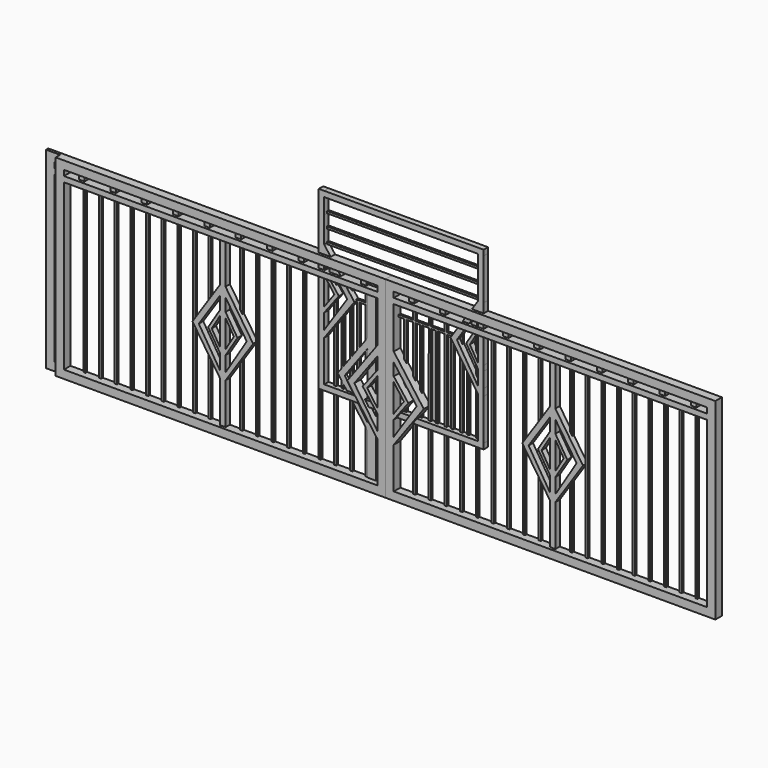
from build123d import *

# Parameters (mm, degrees)
F1_DEPTH  = 76.2
F2_DEPTH  = 25.4
F0_W      = 3048
F0_H      = 1778
F0_W_2    = 50.8
F0_H_2    = 50.8
F3_DEPTH  = 50.8
F4_DEPTH  = 50.8
F0_W_3    = 19.05
F0_H_3    = 1524
F5_DEPTH  = 19.05
F5_TAPER  = -3
F8_DEPTH  = 50.8
F9_DEPTH  = 19.05
F10_DEPTH = 19.05


with BuildPart() as f1:
    # F0 (on Front) → F1 (new body)
    with BuildSketch(Plane.XZ):
        Polygon((3048, 0), (0, 0), (0, -127), (0, -1778), (3048, -1778), align=None)
        Polygon((288.1671190262, -939.8), (76.2, -1257.9814855576), (76.2, -1117.6593963623), (210.9978, -939.8), (76.2, -765.7700244904), (76.2, -652.1689665667), align=None, mode=Mode.SUBTRACT)
        Polygon((76.2, -1069.802350235), (76.2, -813.0455196381), (170.0328290463, -939.8), align=None, mode=Mode.SUBTRACT)
        Polygon((210.9978, -1701.8), (76.2, -1701.8), (76.2, -1322.4239349365), (210.9978, -1137.1291241641), (230.0478, -1110.9427461578), (353.8880646229, -940.7103061676), (230.0478, -772.6639437989), (210.9978, -746.8138439717), (76.2, -563.8985375947), (76.2, -177.8), (210.9978, -177.8), (230.0478, -177.8), (355.7778, -177.8), (374.8278, -177.8), (500.5578, -177.8), (519.6078, -177.8), (645.3378, -177.8), (664.3878, -177.8), (790.1178, -177.8), (809.1678, -177.8), (934.8978, -177.8), (953.9478, -177.8), (1079.6778, -177.8), (1098.7278, -177.8), (1224.4578, -177.8), (1243.5078, -177.8), (1369.2378, -177.8), (1388.2878, -177.8), (1498.6, -177.8), (1549.4, -177.8), (1659.7122, -177.8), (1678.7622, -177.8), (1804.4922, -177.8), (1823.5422, -177.8), (1949.2722, -177.8), (1968.3222, -177.8), (2094.0522, -177.8), (2113.1022, -177.8), (2238.8322, -177.8), (2257.8822, -177.8), (2383.6122, -177.8), (2402.6622, -177.8), (2528.3922, -177.8), (2547.4422, -177.8), (2673.1722, -177.8), (2692.2222, -177.8), (2817.9522, -177.8), (2837.0022, -177.8), (2971.8, -177.8), (2971.8, -1701.8), (2837.0022, -1701.8), (2817.9522, -1701.8), (2692.2222, -1701.8), (2673.1722, -1701.8), (2547.4422, -1701.8), (2528.3922, -1701.8), (2402.6622, -1701.8), (2383.6122, -1701.8), (2257.8822, -1701.8), (2238.8322, -1701.8), (2113.1022, -1701.8), (2094.0522, -1701.8), (1968.3222, -1701.8), (1949.2722, -1701.8), (1823.5422, -1701.8), (1804.4922, -1701.8), (1678.7622, -1701.8), (1659.7122, -1701.8), (1549.4, -1701.8), (1498.6, -1701.8), (1388.2878, -1701.8), (1369.2378, -1701.8), (1243.5078, -1701.8), (1224.4578, -1701.8), (1098.7278, -1701.8), (1079.6778, -1701.8), (953.9478, -1701.8), (934.8978, -1701.8), (809.1678, -1701.8), (790.1178, -1701.8), (664.3878, -1701.8), (645.3378, -1701.8), (519.6078, -1701.8), (500.5578, -1701.8), (374.8278, -1701.8), (352.0028389181, -1701.8), (230.0478, -1701.8), align=None, mode=Mode.SUBTRACT)
        Polygon((196.0372, -127), (76.2, -127), (76.2, -76.2), (196.0372, -76.2), (246.8372, -76.2), (485.5972, -76.2), (536.3972, -76.2), (775.1572, -76.2), (825.9572, -76.2), (1064.7172, -76.2), (1115.5172, -76.2), (1354.2772, -76.2), (1405.0772, -76.2), (1643.8372, -76.2), (1694.6372, -76.2), (1933.3972, -76.2), (1984.1972, -76.2), (2222.9572, -76.2), (2273.7572, -76.2), (2512.5172, -76.2), (2563.3172, -76.2), (2802.0772, -76.2), (2852.8772, -76.2), (2971.8, -76.2), (2971.8, -127), (2852.8772, -127), (2802.0772, -127), (2563.3172, -127), (2512.5172, -127), (2273.7572, -127), (2222.9572, -127), (1984.1972, -127), (1933.3972, -127), (1694.6372, -127), (1643.8372, -127), (1405.0772, -127), (1354.2772, -127), (1115.5172, -127), (1064.7172, -127), (825.9572, -127), (775.1572, -127), (536.3972, -127), (485.5972, -127), (246.8372, -127), align=None, mode=Mode.SUBTRACT)
    extrude(amount=F1_DEPTH)

    # F0 (on Front) → F2 (join)
    with BuildSketch(Plane.XZ):
        Polygon((3048, 0), (0, 0), (0, -127), (0, -1778), (3048, -1778), align=None)
        Polygon((288.1671190262, -939.8), (76.2, -1257.9814855576), (76.2, -1117.6593963623), (210.9978, -939.8), (76.2, -765.7700244904), (76.2, -652.1689665667), align=None, mode=Mode.SUBTRACT)
        Polygon((76.2, -1069.802350235), (76.2, -813.0455196381), (170.0328290463, -939.8), align=None, mode=Mode.SUBTRACT)
        Polygon((210.9978, -1701.8), (76.2, -1701.8), (76.2, -1322.4239349365), (210.9978, -1137.1291241641), (230.0478, -1110.9427461578), (353.8880646229, -940.7103061676), (230.0478, -772.6639437989), (210.9978, -746.8138439717), (76.2, -563.8985375947), (76.2, -177.8), (210.9978, -177.8), (230.0478, -177.8), (355.7778, -177.8), (374.8278, -177.8), (500.5578, -177.8), (519.6078, -177.8), (645.3378, -177.8), (664.3878, -177.8), (790.1178, -177.8), (809.1678, -177.8), (934.8978, -177.8), (953.9478, -177.8), (1079.6778, -177.8), (1098.7278, -177.8), (1224.4578, -177.8), (1243.5078, -177.8), (1369.2378, -177.8), (1388.2878, -177.8), (1498.6, -177.8), (1549.4, -177.8), (1659.7122, -177.8), (1678.7622, -177.8), (1804.4922, -177.8), (1823.5422, -177.8), (1949.2722, -177.8), (1968.3222, -177.8), (2094.0522, -177.8), (2113.1022, -177.8), (2238.8322, -177.8), (2257.8822, -177.8), (2383.6122, -177.8), (2402.6622, -177.8), (2528.3922, -177.8), (2547.4422, -177.8), (2673.1722, -177.8), (2692.2222, -177.8), (2817.9522, -177.8), (2837.0022, -177.8), (2971.8, -177.8), (2971.8, -1701.8), (2837.0022, -1701.8), (2817.9522, -1701.8), (2692.2222, -1701.8), (2673.1722, -1701.8), (2547.4422, -1701.8), (2528.3922, -1701.8), (2402.6622, -1701.8), (2383.6122, -1701.8), (2257.8822, -1701.8), (2238.8322, -1701.8), (2113.1022, -1701.8), (2094.0522, -1701.8), (1968.3222, -1701.8), (1949.2722, -1701.8), (1823.5422, -1701.8), (1804.4922, -1701.8), (1678.7622, -1701.8), (1659.7122, -1701.8), (1549.4, -1701.8), (1498.6, -1701.8), (1388.2878, -1701.8), (1369.2378, -1701.8), (1243.5078, -1701.8), (1224.4578, -1701.8), (1098.7278, -1701.8), (1079.6778, -1701.8), (953.9478, -1701.8), (934.8978, -1701.8), (809.1678, -1701.8), (790.1178, -1701.8), (664.3878, -1701.8), (645.3378, -1701.8), (519.6078, -1701.8), (500.5578, -1701.8), (374.8278, -1701.8), (352.0028389181, -1701.8), (230.0478, -1701.8), align=None, mode=Mode.SUBTRACT)
        Polygon((196.0372, -127), (76.2, -127), (76.2, -76.2), (196.0372, -76.2), (246.8372, -76.2), (485.5972, -76.2), (536.3972, -76.2), (775.1572, -76.2), (825.9572, -76.2), (1064.7172, -76.2), (1115.5172, -76.2), (1354.2772, -76.2), (1405.0772, -76.2), (1643.8372, -76.2), (1694.6372, -76.2), (1933.3972, -76.2), (1984.1972, -76.2), (2222.9572, -76.2), (2273.7572, -76.2), (2512.5172, -76.2), (2563.3172, -76.2), (2802.0772, -76.2), (2852.8772, -76.2), (2971.8, -76.2), (2971.8, -127), (2852.8772, -127), (2802.0772, -127), (2563.3172, -127), (2512.5172, -127), (2273.7572, -127), (2222.9572, -127), (1984.1972, -127), (1933.3972, -127), (1694.6372, -127), (1643.8372, -127), (1405.0772, -127), (1354.2772, -127), (1115.5172, -127), (1064.7172, -127), (825.9572, -127), (775.1572, -127), (536.3972, -127), (485.5972, -127), (246.8372, -127), align=None, mode=Mode.SUBTRACT)
    extrude(amount=F2_DEPTH)

    # F0 (on Front) → F3 (join)
    with BuildSketch(Plane.XZ):
        with Locations((221.4372, -101.6)):
            Rectangle(F0_W_2, F0_H_2)
        with Locations((510.9972, -101.6)):
            Rectangle(F0_W_2, F0_H_2)
        with Locations((800.5572, -101.6)):
            Rectangle(F0_W_2, F0_H_2)
        with Locations((1090.1172, -101.6)):
            Rectangle(F0_W_2, F0_H_2)
        with Locations((1379.6772, -101.6)):
            Rectangle(F0_W_2, F0_H_2)
        with Locations((1669.2372, -101.6)):
            Rectangle(F0_W_2, F0_H_2)
        with Locations((1958.7972, -101.6)):
            Rectangle(F0_W_2, F0_H_2)
        with Locations((2248.3572, -101.6)):
            Rectangle(F0_W_2, F0_H_2)
        with Locations((2537.9172, -101.6)):
            Rectangle(F0_W_2, F0_H_2)
        with Locations((2827.4772, -101.6)):
            Rectangle(F0_W_2, F0_H_2)
    extrude(amount=F3_DEPTH)

    # F0 (on Front) → F4 (join)
    with BuildSketch(Plane.XZ):
        Polygon((1369.2378, -752.0124863089), (1243.5078, -939.8), (1369.2378, -1127.5875136911), (1388.2878, -1156.0401672807), (1498.6, -1320.8), (1498.6, -1701.8), (1549.4, -1701.8), (1549.4, -1320.8), (1659.7122, -1156.0401672807), (1678.7622, -1127.5875136911), (1804.4922, -939.8), (1678.7622, -752.0124863089), (1659.7122, -723.5598327193), (1549.4, -558.8), (1549.4, -177.8), (1498.6, -177.8), (1498.6, -558.8), (1388.2878, -723.5598327193), align=None)
        Polygon((1498.6, -764.1460895538), (1388.2878, -939.8), (1498.6, -1116.0354614258), (1498.6, -1256.357550621), (1302.3867738062, -939.8), (1498.6, -646.7403173447), align=None, mode=Mode.SUBTRACT)
        Polygon((1498.6, -1068.1784152985), (1421.8034963608, -939.8), (1498.6, -811.4215847015), align=None, mode=Mode.SUBTRACT)
        Polygon((1549.4, -764.1460895538), (1549.4, -646.7403173447), (1745.6132261938, -939.8), (1549.4, -1256.357550621), (1549.4, -1116.0354614258), (1659.7122, -939.8), align=None, mode=Mode.SUBTRACT)
        Polygon((1549.4, -1068.1784152985), (1549.4, -811.4215847015), (1626.1965036392, -939.8), align=None, mode=Mode.SUBTRACT)
    extrude(amount=F4_DEPTH)

    # F0 (on Front) → F5 (join)
    with BuildSketch(Plane.XZ):
        Polygon((210.9978, -746.8138439717), (230.0478, -772.6639437989), (230.0478, -177.8), (210.9978, -177.8), align=None)
        Polygon((210.9978, -1137.1291241641), (210.9978, -1701.8), (230.0478, -1701.8), (230.0478, -1110.9427461578), align=None)
        Polygon((353.8880646229, -940.7103061676), (352.0028389181, -1701.8), (374.8278, -1701.8), (374.8278, -177.8), (355.7778, -177.8), align=None)
        with Locations((510.0828, -939.8)):
            Rectangle(F0_W_3, F0_H_3)
        with Locations((654.8628, -939.8)):
            Rectangle(F0_W_3, F0_H_3)
        with Locations((799.6428, -939.8)):
            Rectangle(F0_W_3, F0_H_3)
        with Locations((944.4228, -939.8)):
            Rectangle(F0_W_3, F0_H_3)
        with Locations((1089.2028, -939.8)):
            Rectangle(F0_W_3, F0_H_3)
        Polygon((1224.4578, -177.8), (1224.4578, -1701.8), (1243.5078, -1701.8), (1243.5078, -939.8), (1243.5078, -177.8), align=None)
        Polygon((1369.2378, -1127.5875136911), (1369.2378, -1701.8), (1388.2878, -1701.8), (1388.2878, -1156.0401672807), align=None)
        Polygon((1369.2378, -177.8), (1369.2378, -752.0124863089), (1388.2878, -723.5598327193), (1388.2878, -177.8), align=None)
        Polygon((1678.7622, -177.8), (1659.7122, -177.8), (1659.7122, -723.5598327193), (1678.7622, -752.0124863089), align=None)
        Polygon((1659.7122, -1156.0401672807), (1659.7122, -1701.8), (1678.7622, -1701.8), (1678.7622, -1127.5875136911), align=None)
        Polygon((1804.4922, -939.8), (1804.4922, -1701.8), (1823.5422, -1701.8), (1823.5422, -177.8), (1804.4922, -177.8), align=None)
        with Locations((1958.7972, -939.8)):
            Rectangle(F0_W_3, F0_H_3)
        with Locations((2248.3572, -939.8)):
            Rectangle(F0_W_3, F0_H_3)
        with Locations((2393.1372, -939.8)):
            Rectangle(F0_W_3, F0_H_3)
        with Locations((2537.9172, -939.8)):
            Rectangle(F0_W_3, F0_H_3)
        with Locations((2682.6972, -939.8)):
            Rectangle(F0_W_3, F0_H_3)
        with Locations((2827.4772, -939.8)):
            Rectangle(F0_W_3, F0_H_3)
        with Locations((2103.5772, -939.8)):
            Rectangle(F0_W_3, F0_H_3)
    extrude(amount=F5_DEPTH, taper=F5_TAPER)


with BuildPart() as f2:
    # F0 (on Front) → F2, piece 2 (new body)
    with BuildSketch(Plane.XZ):
        with Locations((-1653.3699964881, -889)):
            Rectangle(F0_W, F0_H)
        Polygon((-340.3677964881, -1137.1291241641), (-205.5699964881, -1322.4239349365), (-205.5699964881, -1701.8), (-340.3677964881, -1701.8), (-359.4177964881, -1701.8), (-481.3728354062, -1701.8), (-504.1977964881, -1701.8), (-629.9277964881, -1701.8), (-648.9777964881, -1701.8), (-774.7077964881, -1701.8), (-793.7577964881, -1701.8), (-919.4877964881, -1701.8), (-938.5377964881, -1701.8), (-1064.2677964881, -1701.8), (-1083.3177964881, -1701.8), (-1209.0477964881, -1701.8), (-1228.0977964881, -1701.8), (-1353.8277964881, -1701.8), (-1372.8777964881, -1701.8), (-1498.6077964881, -1701.8), (-1517.6577964881, -1701.8), (-1627.9699964881, -1701.8), (-1678.7699964881, -1701.8), (-1789.0821964881, -1701.8), (-1808.1321964881, -1701.8), (-1933.8621964881, -1701.8), (-1952.9121964881, -1701.8), (-2078.6421964881, -1701.8), (-2097.6921964881, -1701.8), (-2223.4221964881, -1701.8), (-2242.4721964881, -1701.8), (-2368.2021964881, -1701.8), (-2387.2521964881, -1701.8), (-2512.9821964881, -1701.8), (-2532.0321964881, -1701.8), (-2657.7621964881, -1701.8), (-2676.8121964881, -1701.8), (-2802.5421964881, -1701.8), (-2821.5921964881, -1701.8), (-2947.3221964881, -1701.8), (-2966.3721964881, -1701.8), (-3101.1699964881, -1701.8), (-3101.1699964881, -177.8), (-2966.3721964881, -177.8), (-2947.3221964881, -177.8), (-2821.5921964881, -177.8), (-2802.5421964881, -177.8), (-2676.8121964881, -177.8), (-2657.7621964881, -177.8), (-2532.0321964881, -177.8), (-2512.9821964881, -177.8), (-2387.2521964881, -177.8), (-2368.2021964881, -177.8), (-2242.4721964881, -177.8), (-2223.4221964881, -177.8), (-2097.6921964881, -177.8), (-2078.6421964881, -177.8), (-1952.9121964881, -177.8), (-1933.8621964881, -177.8), (-1808.1321964881, -177.8), (-1789.0821964881, -177.8), (-1678.7699964881, -177.8), (-1627.9699964881, -177.8), (-1517.6577964881, -177.8), (-1498.6077964881, -177.8), (-1372.8777964881, -177.8), (-1353.8277964881, -177.8), (-1228.0977964881, -177.8), (-1209.0477964881, -177.8), (-1083.3177964881, -177.8), (-1064.2677964881, -177.8), (-938.5377964881, -177.8), (-919.4877964881, -177.8), (-793.7577964881, -177.8), (-774.7077964881, -177.8), (-648.9777964881, -177.8), (-629.9277964881, -177.8), (-504.1977964881, -177.8), (-485.1477964881, -177.8), (-359.4177964881, -177.8), (-340.3677964881, -177.8), (-205.5699964881, -177.8), (-205.5699964881, -563.8985375947), (-340.3677964881, -746.8138439717), (-359.4177964881, -772.6639437989), (-483.258061111, -940.7103061676), (-359.4177964881, -1110.9427461578), align=None, mode=Mode.SUBTRACT)
        Polygon((-417.5371155143, -939.8), (-205.5699964881, -652.1689665667), (-205.5699964881, -765.7700244904), (-340.3677964881, -939.8), (-205.5699964881, -1117.6593963623), (-205.5699964881, -1257.9814855576), align=None, mode=Mode.SUBTRACT)
        Polygon((-299.4028255343, -939.8), (-205.5699964881, -813.0455196381), (-205.5699964881, -1069.802350235), align=None, mode=Mode.SUBTRACT)
        Polygon((-3101.1699964881, -127), (-3101.1699964881, -76.2), (-2982.2471964881, -76.2), (-2931.4471964881, -76.2), (-2692.6871964881, -76.2), (-2641.8871964881, -76.2), (-2403.1271964881, -76.2), (-2352.3271964881, -76.2), (-2113.5671964881, -76.2), (-2062.7671964881, -76.2), (-1824.0071964881, -76.2), (-1773.2071964881, -76.2), (-1534.4471964881, -76.2), (-1483.6471964881, -76.2), (-1244.8871964881, -76.2), (-1194.0871964881, -76.2), (-955.3271964881, -76.2), (-904.5271964881, -76.2), (-665.7671964881, -76.2), (-614.9671964881, -76.2), (-376.2071964881, -76.2), (-325.4071964881, -76.2), (-205.5699964881, -76.2), (-205.5699964881, -127), (-325.4071964881, -127), (-376.2071964881, -127), (-614.9671964881, -127), (-665.7671964881, -127), (-904.5271964881, -127), (-955.3271964881, -127), (-1194.0871964881, -127), (-1244.8871964881, -127), (-1483.6471964881, -127), (-1534.4471964881, -127), (-1773.2071964881, -127), (-1824.0071964881, -127), (-2062.7671964881, -127), (-2113.5671964881, -127), (-2352.3271964881, -127), (-2403.1271964881, -127), (-2641.8871964881, -127), (-2692.6871964881, -127), (-2931.4471964881, -127), (-2982.2471964881, -127), align=None, mode=Mode.SUBTRACT)
    extrude(amount=F2_DEPTH)


with BuildPart() as f6_1:
    # F6: instance of F1
    add(f1.part.mirror(Plane.YZ))


with BuildPart() as f8:
    # F7 (on Front) → F8 (new body)
    with BuildSketch(Plane.XZ):
        Polygon((886.6930396151, 518.1709368245), (-586.5069603703, 518.1709368245), (-637.3069603702, 518.1709368248), (-637.3069603702, -1107.4290631752), (886.6930396298, -1107.4290631752), (886.6930396151, -1056.6290631755), (886.69303962, -675.6290631787), (886.6930396151, -611.1866137997), (886.6930396227, -470.8645246045), (886.6930396151, -423.0074784772), (886.6930396267, -166.2506478802), (886.6930396151, -118.9751527325), (886.6930396288, -1.5693805234), (886.6930396151, 86.3709368213), (886.693039635, 467.3709368245), align=None)
        Polygon((-586.5069603699, -424.6314134105), (-586.50696037, -167.8745828136), (-492.6741313237, -294.6290631755), align=None, mode=Mode.SUBTRACT)
        Polygon((-374.5398413439, -294.6290631755), (-586.5069603701, -612.8105487331), (-586.5069603699, -472.4884595378), (-451.7091603701, -294.6290631754), (-586.5069603701, -120.5990876659), (-586.5069603701, -6.9980297422), align=None, mode=Mode.SUBTRACT)
        Polygon((-451.7091603697, -1056.6290631755), (-586.5069603696, -1056.6290631755), (-586.5069603698, -677.252998112), (-451.70916037, -493.1000328573), (-432.65916037, -467.0750236353), (-314.9385648483, -306.2519483558), (-307.9550867601, -296.7115241224), (-314.9627697027, -287.202374326), (-315.1527232202, -287.202374326), (-314.9630779178, -287.2019560901), (-393.5799560315, -180.5219483558), (-407.6183693334, -161.472374326), (-486.2355556622, -54.7919483558), (-500.2739689641, -35.742374326), (-578.8911552929, 70.9380516442), (-586.5069603701, 81.2723992301), (-586.5069603701, 89.987625674), (-586.5069603702, 196.6680516442), (-586.5069603702, 215.717625674), (-586.5069603702, 322.3980516441), (-586.5069603703, 341.447625674), (-586.5069603703, 467.3709368245), (835.893039635, 467.3709368245), (835.8930396333, 343.4368573637), (835.8930396331, 324.3877019187), (835.8930396317, 217.7068573666), (835.8930396315, 198.6577019213), (835.8930396301, 91.9768573666), (835.89303963, 86.3709368243), (826.8923457545, 72.9277019213), (755.4659642967, -33.7531426334), (742.7119197542, -52.8022980787), (671.2855382964, -159.4831426334), (658.5314937539, -178.5322980787), (587.0679343919, -285.268670719), (587.0303742875, -285.3247696502), (580.8008396295, -294.6290631751), (587.2506115052, -304.2622980787), (587.2880608536, -304.3182315872), (587.3255102019, -304.3741650957), (706.530839625, -482.4165768697), (725.5808396243, -510.8692304597), (835.89303962, -675.6290631819), (835.8930396151, -1056.6290631755), (725.5808396195, -1056.6290631755), (706.5308396201, -1056.6290631755), (580.8008396334, -1056.6290631755), (561.7508396259, -1056.6290631755), (436.0208396242, -1056.6290631755), (416.9708396229, -1056.6290631755), (291.240839621, -1056.6290631755), (272.1908396197, -1056.6290631755), (146.4608396154, -1056.6290631755), (127.4108396109, -1056.6290631755), (1.6808396109, -1056.6290631755), (-17.3691603891, -1056.6290631755), (-143.099160389, -1056.6290631755), (-162.149160389, -1056.6290631755), (-287.879160389, -1056.6290631755), (-310.7020499798, -1056.6290631755), (-432.6591603697, -1056.6290631755), align=None, mode=Mode.SUBTRACT)
        Polygon((835.8930396273, -118.9751527319), (725.5808396273, -294.629063178), (835.8930396227, -470.8645246038), (835.8930396209, -611.1866137991), (639.6798134271, -294.629063178), (835.8930396288, -1.5693805227), align=None, mode=Mode.SUBTRACT)
        Polygon((835.8930396233, -423.0074784765), (759.0965359841, -294.629063178), (835.8930396267, -166.2506478796), align=None, mode=Mode.SUBTRACT)
    extrude(amount=F8_DEPTH)

    # F7 (on Front) → F9 (join)
    with BuildSketch(Plane.XZ):
        Polygon((-451.70916037, -493.1000328573), (-451.7091603697, -1056.6290631754), (-432.6591603697, -1056.6290631755), (-432.65916037, -467.0750236353), align=None)
        Polygon((725.5808396243, -510.8692304597), (706.530839625, -482.4165768697), (706.5308396201, -1056.6290631766), (725.5808396195, -1056.6290631755), align=None)
        Polygon((-162.1491603705, -306.0270251887), (-162.149160389, -1056.6290631753), (-143.099160389, -1056.6290631755), (-143.0991603705, -305.9850131154), align=None)
        Polygon((-17.3691603705, -305.7077334319), (-17.3691603891, -1056.6290631753), (1.6808396109, -1056.6290631755), (1.6808396295, -305.6657213586), align=None)
        Polygon((127.4108396296, -305.388441675), (127.4108396109, -1056.6290631784), (146.4608396154, -1056.6290631755), (146.4608396297, -305.3464296018), align=None)
        Polygon((272.1908396298, -305.0691499182), (272.1908396197, -1056.6290631753), (291.240839621, -1056.6290631755), (291.2408396298, -305.0271378449), align=None)
        Polygon((416.9708396298, -304.7498581614), (416.9708396229, -1056.6290631753), (436.0208396242, -1056.6290631755), (436.0208396299, -304.7078460881), align=None)
        Polygon((580.8008396334, -1056.6290631754), (580.80083963, -304.3885543313), (561.7508396299, -304.4305664045), (561.7508396259, -1056.6290631754), align=None)
        Polygon((-307.9895182548, -306.2366232191), (-310.7020499798, -1056.6290631755), (-287.879160389, -1056.6290631755), (-287.8791603705, -306.2482887746), (-287.8791603705, -306.1922726769), align=None)
        Polygon((-314.9385648483, -306.2519483558), (-307.9895182548, -306.2366232191), (-287.8791603705, -306.1922726769), (-162.1491603705, -305.9149929933), (-143.0991603705, -305.8729809201), (-17.3691603705, -305.5957012365), (1.6808396295, -305.5536891632), (127.4108396296, -305.2764094797), (146.4608396297, -305.2343974064), (272.1908396298, -304.9571177228), (291.2408396298, -304.9151056496), (416.9708396298, -304.637825966), (436.0208396299, -304.5958138927), (561.7508396299, -304.3185342092), (580.80083963, -304.2765221359), (587.2506115052, -304.2622980787), (580.8008396299, -294.6290631754), (587.0303742875, -285.3247696502), (587.0679343919, -285.268670719), (-289.7527232202, -287.202374326), (-314.9627697027, -287.202374326), (-307.9550867601, -296.7115241224), align=None)
    extrude(amount=F9_DEPTH)

    # F7 (on Front) → F10 (join)
    with BuildSketch(Plane.XZ):
        Polygon((-586.5069603703, 341.447625674), (-586.5069603702, 322.3980516441), (156.0359997551, 323.4367192513), (225.4866114318, 323.533866628), (294.9372231958, 323.6310140048), (638.0506115052, 324.3877019213), (835.8930396331, 324.3877019187), (835.8930396333, 343.4368573637), (294.0303830334, 342.6790604233), (224.6051018318, 342.5819689094), (155.1798205429, 342.4848773953), (-315.1527232202, 341.447625674), align=None)
        Polygon((-586.5069603702, 215.717625674), (-586.5069603702, 196.6680516442), (156.0360013017, 197.7067192549), (225.4866131237, 197.8038666319), (294.9372252952, 197.9010140094), (638.0506115052, 198.6577019213), (835.8930396315, 198.6577019213), (835.8930396317, 217.7068573666), (294.0303852413, 216.9490604282), (224.6051038656, 216.8519689139), (155.1798224027, 216.7548773994), (-315.1527232202, 215.717625674), align=None)
        Polygon((-586.5069603701, 81.2723992301), (-578.8911552929, 70.9380516442), (157.9324713643, 71.9809016505), (228.8365685714, 72.0812544833), (299.7406656874, 72.181607316), (638.0506115052, 72.9277019213), (826.8923457545, 72.9277019213), (835.89303963, 86.3709368243), (835.8930396301, 91.9768573666), (294.0303852439, 91.2190604282), (224.605103868, 91.1219689139), (155.1798224049, 91.0248773994), (-315.1527232202, 89.987625674), (-586.5069603701, 89.987625674), align=None)
        Polygon((-500.2739689641, -35.742374326), (-486.2355556622, -54.7919483558), (158.0174133522, -53.7489110219), (253.5475527239, -53.5942489455), (349.0776927568, -53.4395868681), (638.0506115052, -52.8022980787), (742.7119197542, -52.8022980787), (755.4659642967, -33.7531426334), (337.2204055146, -34.4156901074), (247.0532099367, -34.5585249718), (156.8860142851, -34.7013598363), (-315.1527232202, -35.742374326), align=None)
        Polygon((-407.6183693334, -161.472374326), (-393.5799560315, -180.5219483558), (158.3027383612, -179.4782817784), (336.5526419443, -179.1411929937), (514.8025455274, -178.8041042089), (638.0506115052, -178.5322980787), (658.5314937539, -178.5322980787), (671.2855382964, -159.4831426334), (466.1289633392, -159.8614005654), (311.2196543558, -160.1470149789), (156.3103452638, -160.4326293927), (-315.1527232202, -161.472374326), align=None)
    extrude(amount=F10_DEPTH)


solid = Compound([f1.part, f2.part, f6_1.part, f8.part])
